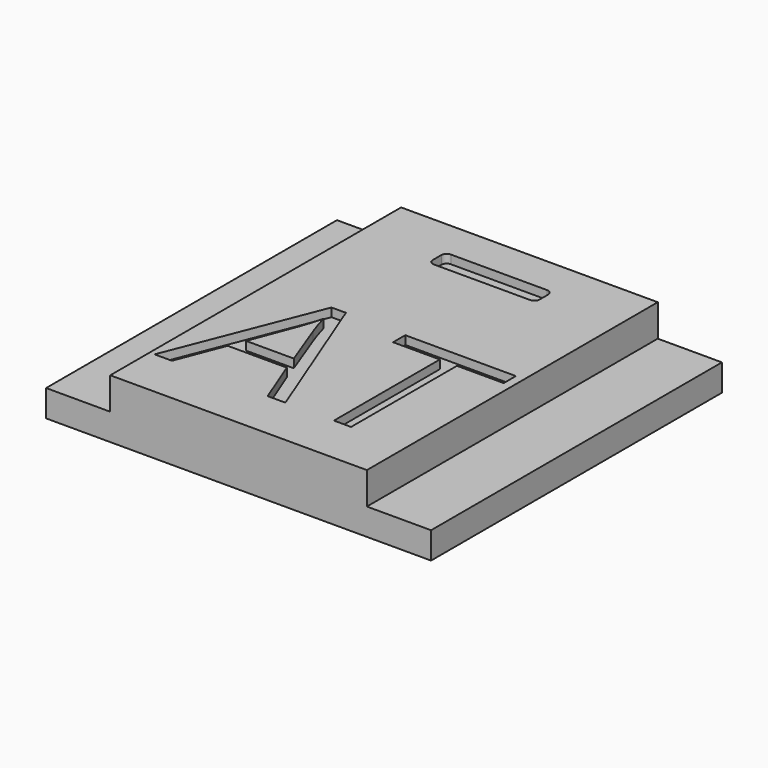
from build123d import *

# Parameters (mm, degrees)
F0_W      = 18
F0_H      = 1.25
F1_DEPTH  = 17
F2_W      = 12
F2_H      = 17
F3_DEPTH  = 1.5
F5_DEPTH  = 3
F6_W      = 4
F6_H      = 1.5
F7_DEPTH  = 0.5
F9_DEPTH  = 25
F11_DEPTH = 0.4


with BuildPart() as f1:
    # F0 (on Front) → F1 (new body)
    with BuildSketch(Plane.XZ):
        Rectangle(F0_W, F0_H)
    extrude(amount=F1_DEPTH)

    # F2 (on face) → F3 (join)
    with BuildSketch(Plane.XY.offset(0.625)):
        with Locations((0, -8.5)):
            Rectangle(F2_W, F2_H)
    extrude(amount=F3_DEPTH)

    # F4 (on face) → F5 (join)
    with BuildSketch(Plane(origin=(0, 0, 0), x_dir=(-1, 0, 0), z_dir=(0, 1, 0))):
        Polygon((-2, 0.375), (-2, -0.625), (0, -0.625), (2, -0.625), (2, 0.375), align=None)
    extrude(amount=F5_DEPTH)

    # F6 (on face) → F7 (cut)
    with BuildSketch(Plane.XY.offset(0.375)):
        with Locations((0, 0.75)):
            Rectangle(F6_W, F6_H)
    extrude(amount=-F7_DEPTH, mode=Mode.SUBTRACT)

    # F8 (on face) → F9 (cut)
    with BuildSketch(Plane(origin=(-2, 0, 0), x_dir=(0, -1, 0), z_dir=(-1, 0, 0))):
        Polygon((-3, 0.375), (-3, -0.125), (-2.5, 0.375), align=None)
    extrude(amount=-F9_DEPTH, mode=Mode.SUBTRACT)

    # F10 (on face) → F11 (cut)
    with BuildSketch(Plane.XY.offset(2.125)):
        with BuildLine():
            Line((0, -2.7756802738), (0, -1.7756802738))
            Line((0, -1.7756802738), (-2.2519526784, -1.7756802738))
            ThreePointArc((-2.2519526784, -1.7756802738), (-2.4273486216, -1.8483316522), (-2.5, -2.0237275953))
            Line((-2.5, -2.0237275953), (-2.5, -2.5276329522))
            ThreePointArc((-2.5, -2.5276329522), (-2.4273486216, -2.7030288953), (-2.2519526784, -2.7756802738))
            Line((-2.2519526784, -2.7756802738), (0, -2.7756802738))
        make_face()
        with BuildLine():
            Line((2.25, -1.7756802738), (0, -1.7756802738))
            Line((0, -1.7756802738), (0, -2.7756802738))
            Line((0, -2.7756802738), (2.2519526784, -2.7756802738))
            ThreePointArc((2.2519526784, -2.7756802738), (2.4273486216, -2.7030288953), (2.5, -2.5276329522))
            Line((2.5, -2.5276329522), (2.5, -2.0256802738))
            ThreePointArc((2.5, -2.0256802738), (2.4267766953, -1.8489035785), (2.25, -1.7756802738))
        make_face()
        Polygon((0, -14.6959666163), (0, -13.8118481482), (-2.3675321166, -7.7671974242), (-3.0425887489, -7.7671974242), (-5.7699987665, -14.6959666163), (-4.9575144977, -14.6959666163), (-4.1087855775, -12.501655013), (-1.3436207146, -12.501655013), (-0.4843204378, -14.6959666163), align=None)
        with BuildLine():
            Line((-2.396225799, -9.6413479402), (-1.592802693, -11.7797823726))
            Line((-1.592802693, -11.7797823726), (-3.8248691415, -11.7797823726))
            Line((-3.8248691415, -11.7797823726), (-3.0138950665, -9.6413479402))
            add(Edge.make_bspline(
                [(-2.7163868863, -8.6461302206), (-2.8205902591, -9.0991883631), (-3.0138950665, -9.6413479402)],
                knots=[0, 0, 0, 1, 1, 1], degree=2))
            add(Edge.make_bspline(
                [(-2.396225799, -9.6413479402), (-2.5517757612, -9.2351058058), (-2.7163868863, -8.6461302206)],
                knots=[0, 0, 0, 1, 1, 1], degree=2))
        make_face(mode=Mode.SUBTRACT)
        Polygon((2.6161074505, -14.6959666163), (3.4180203626, -14.6959666163), (3.4180203626, -8.5087025841), (5.6032708031, -8.5087025841), (5.6032708031, -7.7958911066), (0.43085701, -7.7958911066), (0.43085701, -8.5087025841), (2.6161074505, -8.5087025841), align=None)
        Polygon((0.3462861567, -14.6959666163), (0, -13.8118481482), (0, -14.6959666163), align=None)
    extrude(amount=-F11_DEPTH, mode=Mode.SUBTRACT)


solid = f1.part
